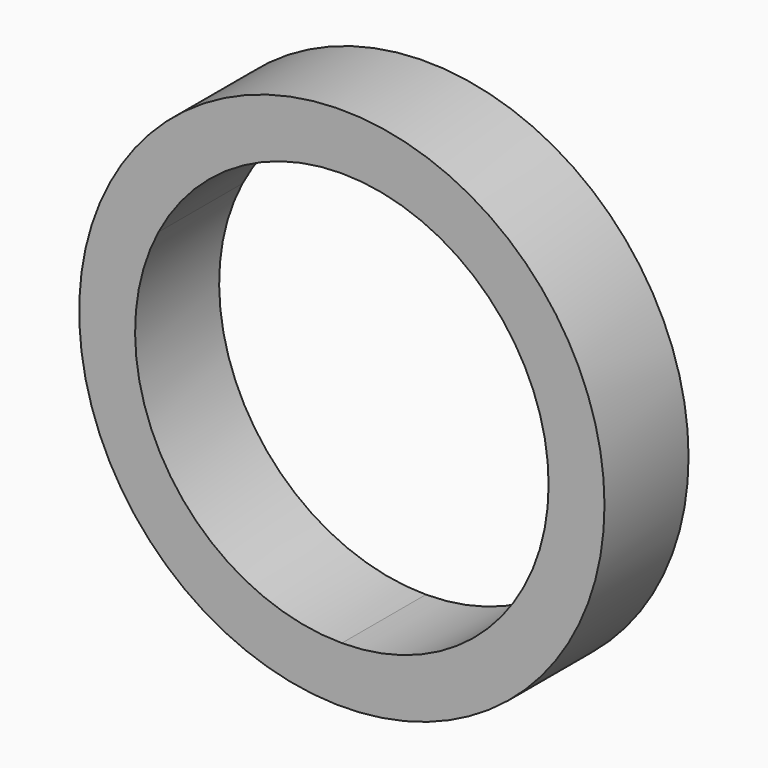
from build123d import *

# Parameters (mm, degrees)
F0_R     = 6.35
F1_DEPTH = 2.54


# Not quite as in the source:
# - a feature names something its author has since deleted; it is built from what else it names


with BuildPart() as f1:
    # F0 (on Front) → F1 (new body)
    with BuildSketch(Plane.XZ):
        with Locations((0, -9.0619377949)):
            Circle(F0_R)
        with BuildLine():
            ThreePointArc((4.4250278693, -6.7369416578), (4.8531244574, -7.864581673), (4.9986476853, -9.0619377949))
            ThreePointArc((4.9986476853, -9.0619377949), (3.534577675, -12.59651547), (0, -14.0605854803))
            ThreePointArc((0, -14.0605854803), (-4.2732397818, -11.6553718984), (-4.434145585, -6.7543781288))
            ThreePointArc((-4.434145585, -6.7543781288), (-0.0098382323, -4.0632997914), (4.4250278693, -6.7369416578))
        make_face(mode=Mode.SUBTRACT)
    extrude(amount=F1_DEPTH)


solid = f1.part
